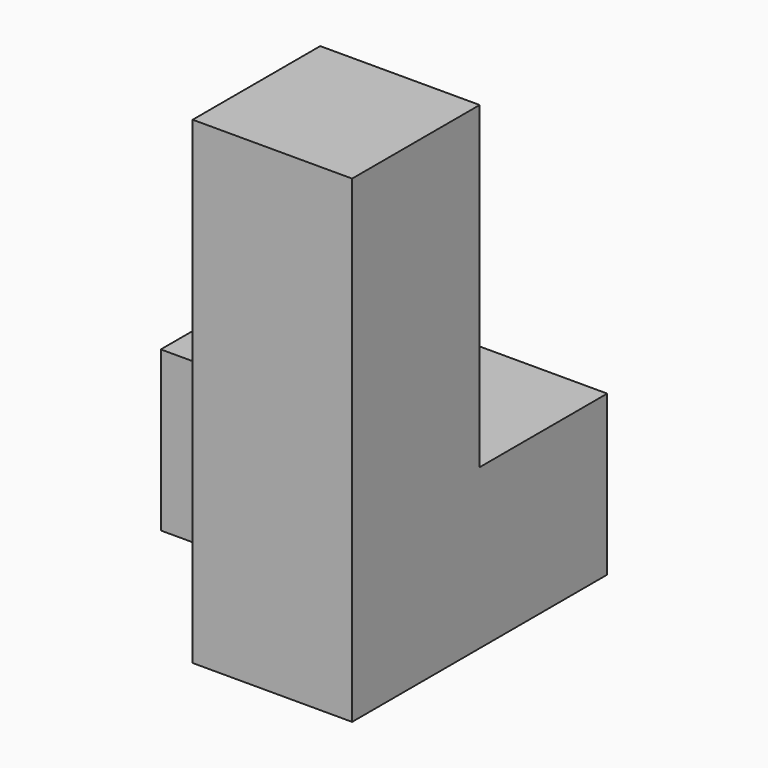
from build123d import *

# Parameters (mm, degrees)
F1_W     = 76.2
F1_H     = 76.2
F2_DEPTH = 228.6
F3_W     = 76.2
F3_H     = 76.2
F4_DEPTH = 76.2
F5_W     = 76.2
F5_H     = 76.2
F6_DEPTH = 76.2


# Not quite as in the source:
# - a variable given as a bare number and used for a length is read in inches; the dataset says mm whatever the document's units were


with BuildPart() as f2:
    # F1 (on Top) → F2 (new body)
    with BuildSketch(Plane.XY):
        Rectangle(F1_W, F1_H)
    extrude(amount=F2_DEPTH)

    # F3 (on face) → F4 (join)
    with BuildSketch(Plane(origin=(0, 38.1, 0), x_dir=(-1, 0, 0), z_dir=(0, 1, 0))):
        with Locations((0, 38.1)):
            Rectangle(F3_W, F3_H)
    extrude(amount=F4_DEPTH)

    # F5 (on face) → F6 (join)
    with BuildSketch(Plane(origin=(-38.1, 0, 0), x_dir=(0, -1, 0), z_dir=(-1, 0, 0))):
        with Locations((-76.2, 38.1)):
            Rectangle(F5_W, F5_H)
    extrude(amount=F6_DEPTH)


solid = f2.part
